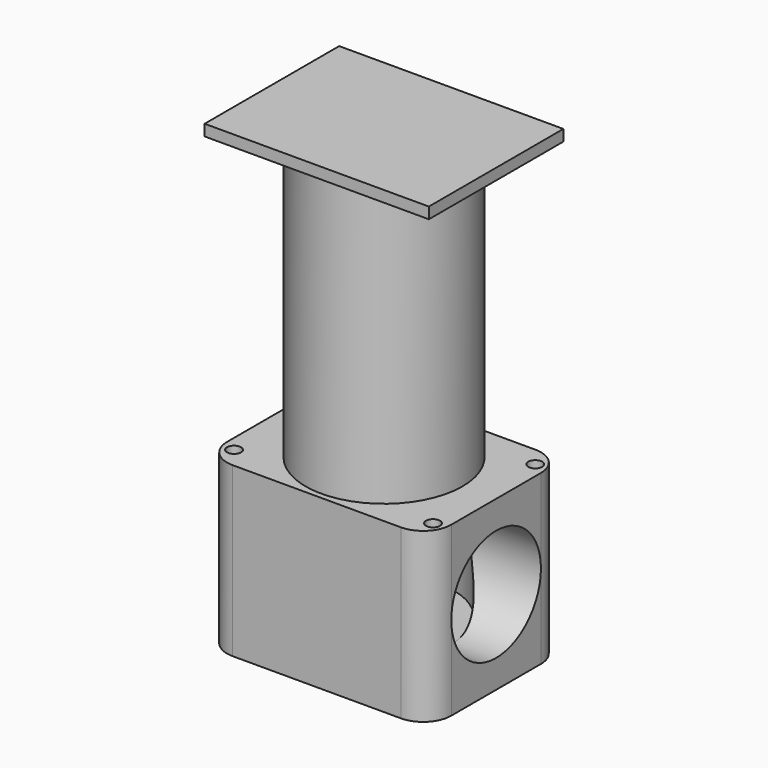
from build123d import *

# Parameters (mm, degrees)
F0_W      = 101.6
F0_H      = 76.2
F0_R      = 3.175
F1_DEPTH  = 203.2
F2_R      = 25.4
F3_DEPTH  = 101.6
F4_R      = 31.75
F5_DEPTH  = 190.5
F6_R      = 12.69999
F7_R      = 3.175
F7_R_2    = 35.56
F8_DEPTH  = 127
F10_W     = 101.6
F10_H     = 76.2
F11_DEPTH = 5.08


# Not quite as in the source:
# - a fillet or chamfer is up to 0.001 mm smaller than in the source, because OpenCascade refuses the exact size


with BuildPart() as f1:
    # F0 (on Top) → F1 (new body)
    with BuildSketch(Plane.XY):
        Rectangle(F0_W, F0_H)
        with Locations((-45.085, -28.5786420731)):
            Circle(F0_R, mode=Mode.SUBTRACT)
        with Locations((45.085, -28.5786420731)):
            Circle(F0_R, mode=Mode.SUBTRACT)
        with Locations((-45.085, 29.3072120343)):
            Circle(F0_R, mode=Mode.SUBTRACT)
        with Locations((45.085, 29.3072120343)):
            Circle(F0_R, mode=Mode.SUBTRACT)
    extrude(amount=F1_DEPTH)

    # F2 (on face) → F3 (cut)
    with BuildSketch(Plane.YZ.offset(50.8)):
        with Locations((0, 38.1)):
            Circle(F2_R)
    extrude(amount=-F3_DEPTH, mode=Mode.SUBTRACT)

    # F4 (on face) → F5 (cut)
    with BuildSketch(Plane.XY.offset(203.2)):
        Circle(F4_R)
    extrude(amount=-F5_DEPTH, mode=Mode.SUBTRACT)

    # F6 (radius 12.7 in the source; OpenCascade refuses exactly that, so slightly less here)
    f6_edges = [f1.edges().sort_by_distance(p)[0] for p in [
        (-50.8, 38.1, 101.6),
        (-50.8, -38.1, 101.6),
        (50.8, -38.1, 101.6),
        (50.8, 38.1, 101.6),
    ]]
    fillet(f6_edges, radius=F6_R)

    # F7 (on face) → F8 (cut)
    with BuildSketch(Plane.XY.offset(203.2)):
        with BuildLine():
            ThreePointArc((50.8, 25.40001), (47.08025905, 34.38025905), (38.10001, 38.1))
            Line((38.10001, 38.1), (-38.10001, 38.1))
            ThreePointArc((-38.10001, 38.1), (-47.08025905, 34.38025905), (-50.8, 25.40001))
            Line((-50.8, 25.40001), (-50.8, -25.40001))
            ThreePointArc((-50.8, -25.40001), (-47.08025905, -34.38025905), (-38.10001, -38.1))
            Line((-38.10001, -38.1), (38.10001, -38.1))
            ThreePointArc((38.10001, -38.1), (47.08025905, -34.38025905), (50.8, -25.40001))
            Line((50.8, -25.40001), (50.8, 25.40001))
        make_face()
        with Locations((-45.085, -28.5786420731)):
            Circle(F7_R, mode=Mode.SUBTRACT)
        with Locations((45.085, -28.5786420731)):
            Circle(F7_R, mode=Mode.SUBTRACT)
        Circle(F7_R_2, mode=Mode.SUBTRACT)
        with Locations((-45.085, 29.3072120343)):
            Circle(F7_R, mode=Mode.SUBTRACT)
        with Locations((45.085, 29.3072120343)):
            Circle(F7_R, mode=Mode.SUBTRACT)
    extrude(amount=-F8_DEPTH, mode=Mode.SUBTRACT)

    # F10 (on offset) → F11 (join)
    with BuildSketch(Plane.XY.offset(203.2)):
        Rectangle(F10_W, F10_H)
    extrude(amount=F11_DEPTH)


solid = f1.part
